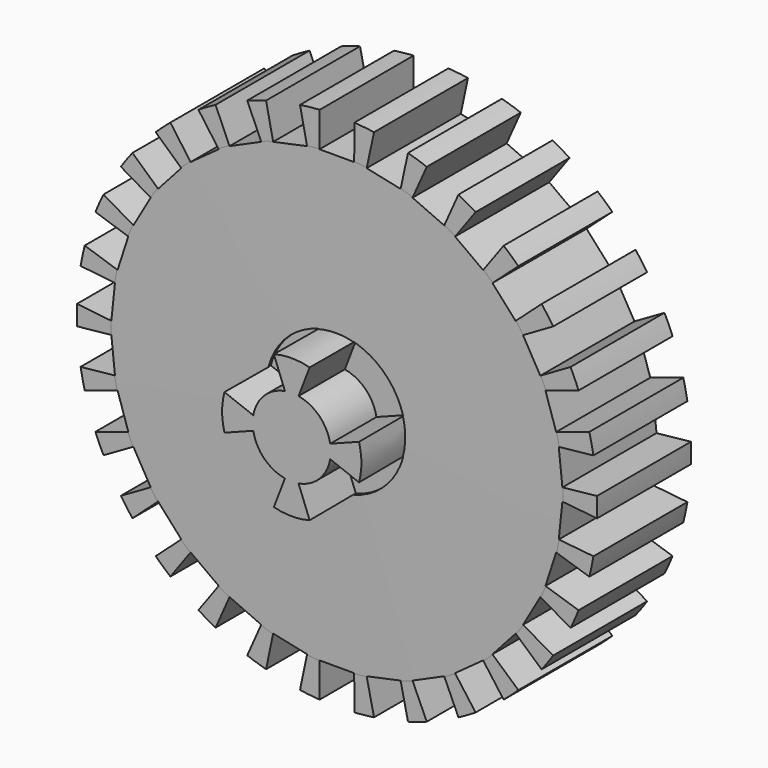
from build123d import *

# Parameters (mm, degrees)
F3_DEPTH        = 27.94
F3_COPIES_COUNT = 30
F6_DEPTH        = 12.7


# Not quite as in the source:
# - a feature of the source that left no trace in its solid (it failed there, or was rolled back) is left out
# - a pattern or mirror of a feature is missing from the dataset's text; its kind, count and spacing are read off the source's solid


with BuildPart() as f1:
    # F0 (on Right) → F1 (revolve)
    with BuildSketch(Plane.YZ):
        Polygon((12.4274313842, 57.15), (12.3881103673, 49.640307582), (38.2248731393, 49.5050253721), (38.2248731393, 57.15), align=None)
        with BuildLine():
            Line((12.1281919494, 0), (38.2248731393, 0))
            Line((38.2248731393, 0), (38.2248731393, 15.2899492557))
            Line((38.2248731393, 15.2899492557), (35.7742973101, 15.2899492557))
            ThreePointArc((35.7742973101, 15.2899492557), (31.2841692496, 17.1498211952), (29.4242973101, 21.6399492557))
            Line((29.4242973101, 21.6399492557), (29.4242973101, 35.5100507443))
            ThreePointArc((29.4242973101, 35.5100507443), (31.2841692496, 40.0001788048), (35.7742973101, 41.8600507443))
            Line((35.7742973101, 41.8600507443), (38.2248731393, 41.8600507443))
            Line((38.2248731393, 41.8600507443), (38.2248731393, 49.5050253721))
            Line((38.2248731393, 49.5050253721), (12.3881103673, 49.640307582))
            Line((12.3881103673, 49.640307582), (12.1281919494, 15.2264456108))
            Line((12.1281919494, 15.2264456108), (0, 15.2899492557))
            Line((0, 15.2899492557), (0, 0))
            Line((0, 0), (12.1281919494, 0))
        make_face()
    revolve(axis=Axis((0, 25.1765325443, 0), (0, -1, 0)))

    # F2 (on face) → F3 (cut)
    with BuildSketch(Plane(origin=(0, 38.2248731393, 0), x_dir=(-1, 0, 0), z_dir=(0, 1, 0))):
        with BuildLine():
            Line((3.81, 49.4028585744), (3.81, 57.0228585744))
            ThreePointArc((3.81, 57.0228585744), (0, 57.15), (-3.81, 57.0228585744))
            Line((-3.81, 57.0228585744), (-3.81, 49.4028585744))
            Line((-3.81, 49.4028585744), (0, 49.4028585744))
            Line((0, 49.4028585744), (3.81, 49.4028585744))
        make_face()
    f3 = extrude(amount=-F3_DEPTH, mode=Mode.SUBTRACT)

    # F3_copies: F3 ×30 about axis
    f3_copies_axis = Axis((0, 0, 0), (0, 1, 0))
    for i in range(1, F3_COPIES_COUNT):
        add(f3.rotate(f3_copies_axis, i * 360 / F3_COPIES_COUNT), mode=Mode.SUBTRACT)

    # F5 (on face) → F6 (cut)
    with BuildSketch(Plane.XZ):
        with BuildLine():
            Line((-1.496441, 8.4486927509), (-3.9260018, 14.7773156598))
            ThreePointArc((-3.9260018, 14.7773156598), (-10.8116268027, 10.8116268027), (-14.7773156598, 3.9260018))
            Line((-14.7773156598, 3.9260018), (-8.4486927509, 1.496441))
            ThreePointArc((-8.4486927509, 1.496441), (-6.0671140118, 6.0671140118), (-1.496441, 8.4486927509))
        make_face()
        with BuildLine():
            ThreePointArc((14.7773156598, 3.9260018), (10.8116268027, 10.8116268027), (3.9260018, 14.7773156598))
            Line((3.9260018, 14.7773156598), (1.496441, 8.4486927509))
            ThreePointArc((1.496441, 8.4486927509), (6.0671140118, 6.0671140118), (8.4486927509, 1.496441))
            Line((8.4486927509, 1.496441), (14.7773156598, 3.9260018))
        make_face()
        with BuildLine():
            Line((-8.4486927509, -1.496441), (-14.7773156598, -3.9260018))
            ThreePointArc((-14.7773156598, -3.9260018), (-10.8116268027, -10.8116268027), (-3.9260018, -14.7773156598))
            Line((-3.9260018, -14.7773156598), (-1.496441, -8.4486927509))
            ThreePointArc((-1.496441, -8.4486927509), (-6.0671140118, -6.0671140118), (-8.4486927509, -1.496441))
        make_face()
        with BuildLine():
            ThreePointArc((3.9260018, -14.7773156598), (10.8116268027, -10.8116268027), (14.7773156598, -3.9260018))
            Line((14.7773156598, -3.9260018), (8.4486927509, -1.496441))
            ThreePointArc((8.4486927509, -1.496441), (6.0671140118, -6.0671140118), (1.496441, -8.4486927509))
            Line((1.496441, -8.4486927509), (3.9260018, -14.7773156598))
        make_face()
    extrude(amount=-F6_DEPTH, mode=Mode.SUBTRACT)


solid = f1.part
